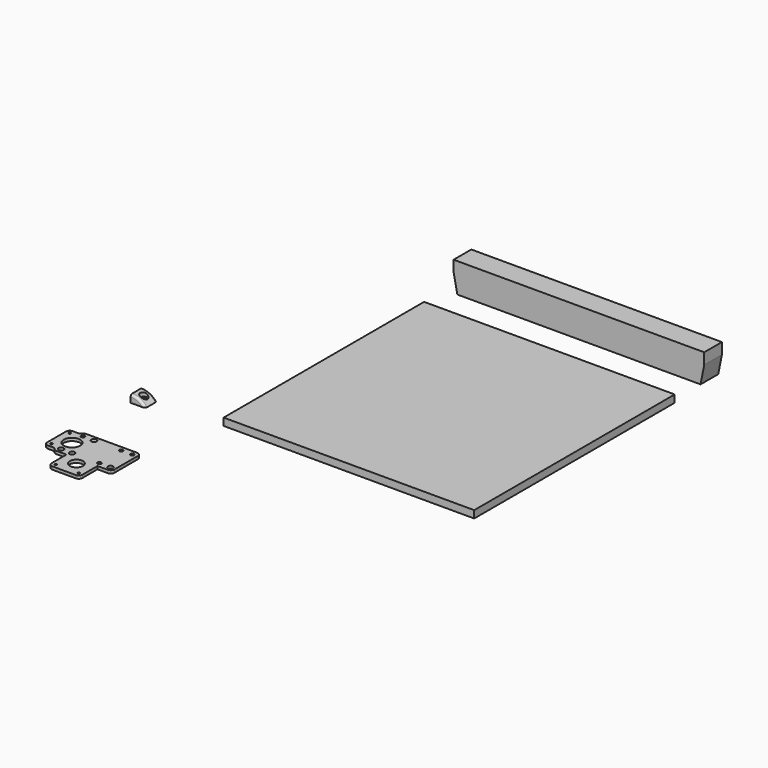
from build123d import *

# Parameters (mm, degrees)
F0_R          = 3.555
F0_R_2        = 1.5
F0_R_3        = 9
F0_R_4        = 11.2
F0_R_5        = 2.5
F1_DEPTH      = 4
F0_W          = 340
F0_H          = 340
F2_DEPTH      = 10
F6_DEPTH      = 39.1
F6_DEPTH_BACK = 25
F0_W_2        = 20
F0_H_2        = 20
F0_R_6        = 5
F8_DEPTH      = 10
F9_DEPTH      = 4
F11_DEPTH     = 25
F12_R         = 3
F13_D         = 2.5
F13_DEPTH     = 8
F13_TIP       = 0.7510757738
F0_H_3        = 30
F14_DEPTH     = 40
F15_SIZE2     = 25
F15_SIZE      = 5


# Not quite as in the source:
# - a feature of the source that left no trace in its solid (it failed there, or was rolled back) is left out
# - a feature names something its author has since deleted; it is built from what else it names


with BuildPart() as f1:
    # F0 (on Top) → F1 (new body)
    with BuildSketch(Plane.XY):
        with BuildLine():
            Line((35, 25), (-35, 25))
            ThreePointArc((-35, 25), (-38.1622776602, 23.8729833462), (-39.8989794856, 21))
            Line((-39.8989794856, 21), (-49.5, 21))
            ThreePointArc((-49.5, 21), (-53.0355339059, 19.5355339059), (-54.5, 16))
            Line((-54.5, 16), (-54.5, -16))
            ThreePointArc((-54.5, -16), (-53.0355339059, -19.5355339059), (-49.5, -21))
            Line((-49.5, -21), (-39.8989794856, -21))
            ThreePointArc((-39.8989794856, -21), (-38.1622776602, -23.8729833462), (-35, -25))
            Line((-35, -25), (-21, -25))
            Line((-21, -25), (-21, -50.5))
            ThreePointArc((-21, -50.5), (-19.5355339059, -54.0355339059), (-16, -55.5))
            Line((-16, -55.5), (16, -55.5))
            ThreePointArc((16, -55.5), (19.5355339059, -54.0355339059), (21, -50.5))
            Line((21, -50.5), (21, -25))
            Line((21, -25), (35, -25))
            ThreePointArc((35, -25), (38.5355339059, -23.5355339059), (40, -20))
            Line((40, -20), (40, 20))
            ThreePointArc((40, 20), (38.5355339059, 23.5355339059), (35, 25))
        make_face()
        with Locations((-33.5, -18.5)):
            Circle(F0_R, mode=Mode.SUBTRACT)
        with Locations((-15.5, -50)):
            Circle(F0_R_2, mode=Mode.SUBTRACT)
        with BuildLine():
            ThreePointArc((-21, -15.9725457472), (-17.1305977581, -15.2193350522), (-14.945, -18.5))
            ThreePointArc((-14.945, -18.5), (-17.1305977581, -21.7806649478), (-21, -21.0274542528))
            ThreePointArc((-21, -21.0274542528), (-22.055, -18.5), (-21, -15.9725457472))
        make_face(mode=Mode.SUBTRACT)
        with Locations((0, -34.5)):
            Circle(F0_R_3, mode=Mode.SUBTRACT)
        with Locations((-49, -15.5)):
            Circle(F0_R_2, mode=Mode.SUBTRACT)
        with Locations((-33.5, 0)):
            Circle(F0_R_4, mode=Mode.SUBTRACT)
        with Locations((-49, 15.5)):
            Circle(F0_R_2, mode=Mode.SUBTRACT)
        with Locations((-33.5, 18.5)):
            Circle(F0_R_5, mode=Mode.SUBTRACT)
        with Locations((-18.5, 18.5)):
            Circle(F0_R, mode=Mode.SUBTRACT)
        with Locations((15.5, -50)):
            Circle(F0_R_2, mode=Mode.SUBTRACT)
        with Locations((18.5, -18.5)):
            Circle(F0_R_5, mode=Mode.SUBTRACT)
        with Locations((33.5, -18.5)):
            Circle(F0_R, mode=Mode.SUBTRACT)
        with Locations((18.5, 18.5)):
            Circle(F0_R_5, mode=Mode.SUBTRACT)
        with Locations((33.5, 18.5)):
            Circle(F0_R_5, mode=Mode.SUBTRACT)
    extrude(amount=F1_DEPTH)

    # F5 (on Front) → F6 (cut, two sides)
    with BuildSketch(Plane.XZ) as f6_sk:
        with BuildLine():
            ThreePointArc((302.9023957253, 6.4145649905), (305.9114714076, 3.7905540573), (307.1651339531, 0))
            Line((307.1651339531, 0), (307.1651339531, 41.5010216767))
            Line((307.1651339531, 41.5010216767), (278.5302054882, 41.5010216767))
            ThreePointArc((278.5302054882, 41.5010216767), (286.2334403864, 20.8438533005), (302.9023957253, 6.4145649905))
        make_face()
    extrude(amount=F6_DEPTH, mode=Mode.SUBTRACT)
    extrude(f6_sk.sketch, amount=-F6_DEPTH_BACK, mode=Mode.SUBTRACT)


with BuildPart() as f2:
    # F0 (on Top) → F2 (new body)
    with BuildSketch(Plane.XY):
        with Locations((233.1544440985, 306.2372636795)):
            Rectangle(F0_W, F0_H)
    extrude(amount=F2_DEPTH)

    # F13
    with Locations(Plane(origin=(0, 0, 0), x_dir=(1, 0, 0), z_dir=(0, 0, -1))):
        with Locations((73.1544440985, -151.2372636795), (73.1544440985, -191.2372636795), (73.1544440985, -306.2372636795), (72.901290132, -421.2380647742), (73.1544440985, -461.2372636795), (393.1544440985, -151.2372636795), (393.1544440985, -461.2372636795), (233.1544440985, -461.2372636795), (233.1544440985, -151.2372636795)):
            Hole(F13_D / 2, depth=F13_DEPTH)
            with Locations((0, 0, -(F13_DEPTH + F13_TIP / 2))):  # 118° drill point
                Cone(0, F13_D / 2, F13_TIP, mode=Mode.SUBTRACT)


with BuildPart() as f8:
    # F0 (on Top) → F8 (new body)
    with BuildSketch(Plane.XY):
        with Locations((-36.9331801683, 126.1065623164)):
            Rectangle(F0_W_2, F0_H_2)
        with Locations((-36.9331801683, 126.1065623164)):
            Circle(F0_R_6, mode=Mode.SUBTRACT)
    extrude(amount=F8_DEPTH)

    # F0 (on Top) → F9 (join)
    with BuildSketch(Plane.XY):
        with Locations((-36.9331801683, 126.1065623164)):
            Circle(F0_R_6)
        with Locations((-36.9331801683, 126.1065623164)):
            Circle(F0_R_5, mode=Mode.SUBTRACT)
    extrude(amount=F9_DEPTH)

    # F10 (on face) → F11 (cut)
    with BuildSketch(Plane.XZ.offset(-116.1065623164)):
        with BuildLine():
            ThreePointArc((-46.9331801683, 10), (-35.7528402808, 7.360679775), (-26.9331801683, 0))
            Line((-26.9331801683, 0), (-26.9331801683, 10))
            Line((-26.9331801683, 10), (-46.9331801683, 10))
        make_face()
    extrude(amount=-F11_DEPTH, mode=Mode.SUBTRACT)

    # F12
    f12_edges = [f8.edges().sort_by_distance(p)[0] for p in [
        (-35.75284, 116.106562, 7.36068),
        (-35.75284, 136.106562, 7.36068),
    ]]
    fillet(f12_edges, radius=F12_R)


with BuildPart() as f14:
    # F0 (on Top) → F14 (new body)
    with BuildSketch(Plane.XY):
        with Locations((233.1544440985, 541.3095498085)):
            Rectangle(F0_W, F0_H_3)
    extrude(amount=F14_DEPTH)

    # F15
    f15_edges = [f14.edges().sort_by_distance(p)[0] for p in [
        (63.154444, 541.30955, 0),
        (403.154444, 541.30955, 0),
    ]]
    f15_side = f14.faces().sort_by_distance((233.154444, 541.30955, 0))[0]
    chamfer(f15_edges, length=F15_SIZE, length2=F15_SIZE2, reference=f15_side)


solid = Compound([f1.part, f2.part, f8.part, f14.part])
